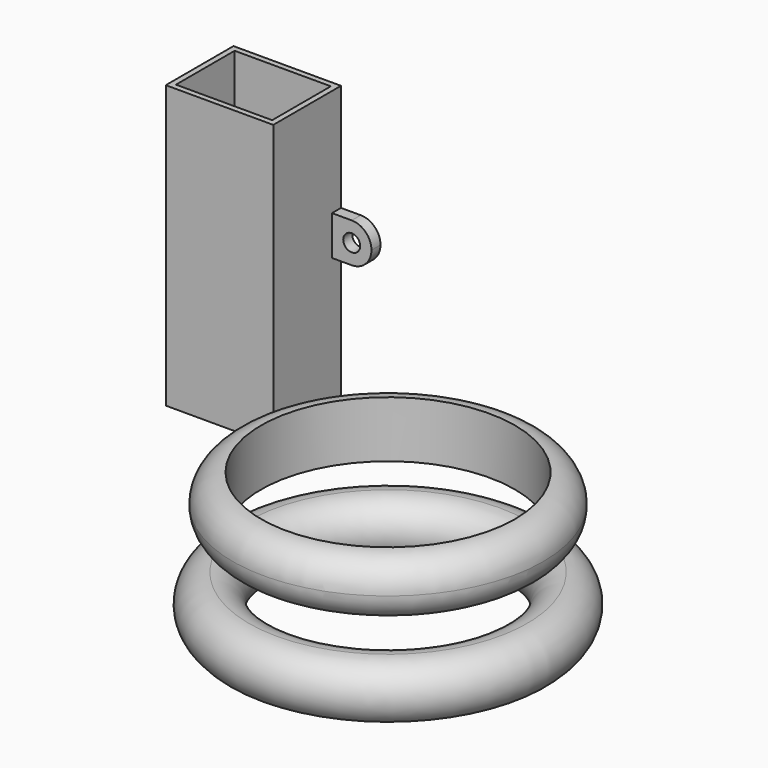
from build123d import *

# Parameters (mm, degrees)
F0_W      = 19.05
F0_H      = 15
F1_DEPTH  = 50
F2_T      = -1
F3_W      = 2
F3_H      = 7
F4_DEPTH  = 7
F5_R      = 3.49999
F6_W      = 2
F6_H      = 7
F7_DEPTH  = 7
F8_R      = 3.49999
F9_R      = 1.5
F10_DEPTH = 25
F11_R     = 27.5
F11_R_2   = 22.5
F12_DEPTH = 10
F13_R     = 4.99999
F18_DEPTH = 2


# Not quite as in the source:
# - a fillet or chamfer is up to 0.001 mm smaller than in the source, because OpenCascade refuses the exact size


with BuildPart() as f1:
    # F0 (on Top) → F1 (new body)
    with BuildSketch(Plane.XY):
        with Locations((-38.9581184149, 18.8712536544)):
            Rectangle(F0_W, F0_H)
    extrude(amount=F1_DEPTH)

    # F2
    f2_openings = [f1.faces().sort_by_distance(p)[0] for p in [
        (-38.958118, 18.871254, 50),
        (-38.958118, 18.871254, 0),
    ]]
    offset(amount=F2_T, openings=f2_openings)

    # F3 (on face) → F4 (join)
    with BuildSketch(Plane(origin=(-48.4831184149, 0, 0), x_dir=(0, -1, 0), z_dir=(-1, 0, 0))):
        with Locations((-25.3712536544, 27.45)):
            Rectangle(F3_W, F3_H)
    extrude(amount=F4_DEPTH)

    # F5 (radius 3.5 in the source; OpenCascade refuses exactly that, so slightly less here)
    f5_edges = [f1.edges().sort_by_distance(p)[0] for p in [
        (-55.483118, 25.371254, 30.95),
        (-55.483118, 25.371254, 23.95),
    ]]
    fillet(f5_edges, radius=F5_R)

    # F6 (on face) → F7 (join)
    with BuildSketch(Plane.YZ.offset(-29.4331184149)):
        with Locations((25.3712536544, 27.45)):
            Rectangle(F6_W, F6_H)
    extrude(amount=F7_DEPTH)

    # F8 (radius 3.5 in the source; OpenCascade refuses exactly that, so slightly less here)
    f8_edges = [f1.edges().sort_by_distance(p)[0] for p in [
        (-22.433118, 25.371254, 30.95),
        (-22.433118, 25.371254, 23.95),
    ]]
    fillet(f8_edges, radius=F8_R)

    # F9 (on face) → F10 (cut)
    with BuildSketch(Plane(origin=(0, 26.3712536544, 0), x_dir=(-1, 0, 0), z_dir=(0, 1, 0))):
        with Locations((25.9331184149, 27.45)):
            Circle(F9_R)
        with Locations((51.9831184149, 27.45)):
            Circle(F9_R)
    extrude(amount=-F10_DEPTH, mode=Mode.SUBTRACT)


with BuildPart() as f12:
    # F11 (on Top) → F12 (new body)
    with BuildSketch(Plane.XY):
        Circle(F11_R)
        Circle(F11_R_2, mode=Mode.SUBTRACT)
    extrude(amount=F12_DEPTH)

    # F13 (radius 5 in the source; OpenCascade refuses exactly that, so slightly less here)
    f13_edges = [f12.edges().sort_by_distance(p)[0] for p in [
        (-27.5, 0, 10),
        (-27.5, 0, 0),
    ]]
    fillet(f13_edges, radius=F13_R)


with BuildPart() as f16:
    # F14 (on Right) → F16 (revolve)
    with BuildSketch(Plane.YZ):
        with BuildLine():
            ThreePointArc((-21.586292201, -14.5089704435), (-19.94302217, -8.9419837234), (-24.6695839419, -5.5728159699))
            ThreePointArc((-24.6695839419, -5.5728159699), (-29.3961457139, -8.9419837234), (-27.7528756829, -14.5089704435))
            Line((-27.7528756829, -14.5089704435), (-24.6695839419, -14.5089704435))
            Line((-24.6695839419, -14.5089704435), (-21.586292201, -14.5089704435))
        make_face()
        with BuildLine():
            ThreePointArc((-24.6695839419, -14.0728159699), (-28.1695839419, -10.5728159699), (-24.6695839419, -7.0728159699))
            ThreePointArc((-24.6695839419, -7.0728159699), (-22.1947102078, -8.0979422357), (-21.1695839419, -10.5728159699))
            ThreePointArc((-21.1695839419, -10.5728159699), (-22.1947102078, -13.047689704), (-24.6695839419, -14.0728159699))
        make_face(mode=Mode.SUBTRACT)
    revolve(axis=Axis((0, 0, 0), (0, 0, 1)))

    # F17 (on face) → F18 (cut)
    with BuildSketch(Plane(origin=(0, 0, -14.5089704435), x_dir=(1, 0, 0), z_dir=(0, 0, -1))):
        with BuildLine():
            add(Edge.make_bspline(
                [(-18.5693163885, 11.0067479234), (-19.5145440214, 11.8822279008), (-20.2784297379, 12.748853493), (-20.7013416556, 13.4180037833)],
                knots=[0, 0, 0, 0, 0.2849335845, 0.2849335845, 0.2849335845, 0.2849335845], degree=3))
            Line((-18.5693163885, 11.0067479234), (-16.3423760275, 9.3934229103))
            Line((-16.3423760275, 9.3934229103), (-14.6021316763, 11.9121490585))
            Line((-14.6021316763, 11.9121490585), (-16.8639985197, 13.4749235587))
            add(Edge.make_bspline(
                [(-19.8941943816, 14.5879882704), (-19.1286458444, 14.4140509933), (-18.0515904183, 13.998916464), (-16.8639985197, 13.4749235587)],
                knots=[0.7146788605, 0.7146788605, 0.7146788605, 0.7146788605, 1, 1, 1, 1], degree=3))
            ThreePointArc((-19.8941943816, 14.5879882704), (-20.3061961593, 14.0088104209), (-20.7013416556, 13.4180037833))
        make_face()
        with BuildLine():
            add(Edge.make_bspline(
                [(-20.7013416556, 13.4180037833), (-21.0205534128, 13.9230750074), (-21.2702357528, 14.7075006253), (-20.4702017813, 14.7188606498), (-19.8941943816, 14.5879882704)],
                knots=[0.2849335845, 0.2849335845, 0.2849335845, 0.2849335845, 0.5, 0.7146788605, 0.7146788605, 0.7146788605, 0.7146788605], degree=3))
            ThreePointArc((-20.7013416556, 13.4180037833), (-20.3061961593, 14.0088104209), (-19.8941943816, 14.5879882704))
        make_face()
    extrude(amount=-F18_DEPTH, mode=Mode.SUBTRACT)


solid = Compound([f1.part, f12.part, f16.part])
